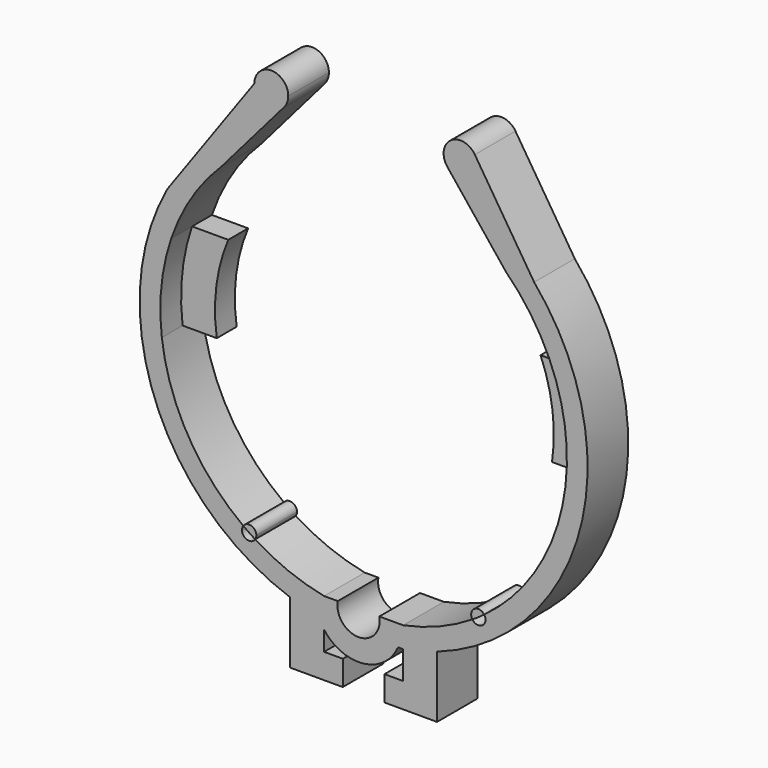
from build123d import *

# Parameters (mm, degrees)
F1_DEPTH = 4.5
F2_DEPTH = 2.2


with BuildPart() as f1:
    # F0 (on Front) → F1 (new body)
    with BuildSketch(Plane.XZ):
        with BuildLine():
            Line((-12.5982642878, 12.8562722799), (-17.3673227921, 9.5716989334))
            ThreePointArc((-17.3673227921, 9.5716989334), (-18.5128661298, -7.1073981948), (-6.5, -18.7347623801))
            ThreePointArc((-6.5, -18.7347623801), (-5.0153521077, -19.1856082696), (-3.5, -19.5189989866))
            Line((-3.5, -19.5189989866), (-3.5, -17.656443583))
            ThreePointArc((-3.5, -17.656443583), (-6.6633813431, -16.7212245089), (-9.6029714558, -15.2244191751))
            ThreePointArc((-9.6029714558, -15.2244191751), (-10.4915008811, -15.4010270522), (-10.6524086102, -14.5095206951))
            ThreePointArc((-10.6524086102, -14.5095206951), (-15.5351423919, -9.0917188069), (-17.8673478305, -2.1812568633))
            ThreePointArc((-17.8673478305, -2.1812568633), (-17.9030269403, 1.8659116739), (-17.033561821, 5.8187431367))
            ThreePointArc((-17.033561821, 5.8187431367), (-15.2280328258, 9.5972400332), (-12.5982642878, 12.8562722799))
        make_face()
        with BuildLine():
            Line((-9.6738959998, 20.2858578414), (-17.3673227921, 9.5716989334))
            Line((-17.3673227921, 9.5716989334), (-12.5982642878, 12.8562722799))
            Line((-12.5982642878, 12.8562722799), (-7.0377798874, 19.3064497655))
            ThreePointArc((-7.0377798874, 19.3064497655), (-8.696306677, 18.8797685539), (-9.6738959998, 20.2858578414))
        make_face()
        with BuildLine():
            ThreePointArc((-3.5, -19.5189989866), (-5.0153521077, -19.1856082696), (-6.5, -18.7347623801))
            Line((-6.5, -18.7347623801), (-6.5, -24.2152123027))
            Line((-6.5, -24.2152123027), (-1.8481902329, -24.2152123027))
            Line((-1.8481902329, -24.2152123027), (-1.8312213279, -22.0041828084))
            Line((-1.8312213279, -22.0041828084), (-3.5, -22.0041828084))
            Line((-3.5, -22.0041828084), (-3.5, -20.2840574679))
            ThreePointArc((-3.5, -20.2840574679), (-3.7451179805, -19.9145035902), (-3.945689667, -19.5189989866))
            Line((-3.945689667, -19.5189989866), (-3.5, -19.5189989866))
        make_face()
        with BuildLine():
            ThreePointArc((-6.6738959998, 20.2858578414), (-8.1738959998, 21.7858578414), (-9.6738959998, 20.2858578414))
            ThreePointArc((-9.6738959998, 20.2858578414), (-8.696306677, 18.8797685539), (-7.0377798874, 19.3064497655))
            ThreePointArc((-7.0377798874, 19.3064497655), (-6.7678067123, 19.7634471641), (-6.6738959998, 20.2858578414))
        make_face()
        with BuildLine():
            Line((-3.5, -17.656443583), (-3.5, -19.5189989866))
            Line((-3.5, -19.5189989866), (-3.5, -20.2840574679))
            ThreePointArc((-3.5, -20.2840574679), (-0.0064092924, -21.7831240851), (3.0474594497, -19.5189989866))
            Line((3.0474594497, -19.5189989866), (3.5, -19.5189989866))
            Line((3.5, -19.5189989866), (3.5, -17.656443583))
            Line((3.5, -17.656443583), (3.3503894936, -17.656443583))
            Line((3.3503894936, -17.656443583), (2.321347558, -17.656443583))
            Line((2.321347558, -17.656443583), (1.3912129293, -17.656443583))
            ThreePointArc((1.3912129293, -17.656443583), (-0.4491151087, -19.8654973153), (-2.2894431467, -17.656443583))
            Line((-2.2894431467, -17.656443583), (-2.854652442, -17.656443583))
            Line((-2.854652442, -17.656443583), (-3.5, -17.656443583))
        make_face()
        with BuildLine():
            Line((-3.5, -20.2840574679), (-3.5, -19.5189989866))
            Line((-3.5, -19.5189989866), (-3.945689667, -19.5189989866))
            ThreePointArc((-3.945689667, -19.5189989866), (-3.7451179805, -19.9145035902), (-3.5, -20.2840574679))
        make_face()
        with BuildLine():
            ThreePointArc((6.5, -18.7347623801), (5.0153521077, -19.1856082696), (3.5, -19.5189989866))
            Line((3.5, -19.5189989866), (3.5, -22.0041828084))
            Line((3.5, -22.0041828084), (1.8481902329, -22.0041828084))
            Line((1.8481902329, -22.0041828084), (1.8312213279, -24.2152123027))
            Line((1.8312213279, -24.2152123027), (6.5, -24.2152123027))
            Line((6.5, -24.2152123027), (6.5, -18.7347623801))
        make_face()
        with BuildLine():
            Line((3.5, -17.656443583), (3.5, -19.5189989866))
            ThreePointArc((3.5, -19.5189989866), (5.0153521077, -19.1856082696), (6.5, -18.7347623801))
            ThreePointArc((6.5, -18.7347623801), (19.1342526058, -5.2078497151), (15.0982642878, 12.8562722799))
            Line((15.0982642878, 12.8562722799), (12.5982642878, 12.8562722799))
            ThreePointArc((12.5982642878, 12.8562722799), (15.2280328258, 9.5972400332), (17.033561821, 5.8187431367))
            ThreePointArc((17.033561821, 5.8187431367), (17.9030269403, 1.8659116739), (17.8673478305, -2.1812568633))
            ThreePointArc((17.8673478305, -2.1812568633), (15.5430874553, -9.0781293423), (10.6777704031, -14.4908667518))
            ThreePointArc((10.6777704031, -14.4908667518), (10.7649831427, -14.665553176), (10.795, -14.8584790608))
            ThreePointArc((10.795, -14.8584790608), (10.3422246395, -15.4667710801), (9.6295852574, -15.2075996715))
            ThreePointArc((9.6295852574, -15.2075996715), (6.6780020503, -16.7153907707), (3.5, -17.656443583))
        make_face()
        with BuildLine():
            Line((12.5982642878, 12.8562722799), (15.0982642878, 12.8562722799))
            Line((15.0982642878, 12.8562722799), (9.8459355165, 21.0923907272))
            ThreePointArc((9.8459355165, 21.0923907272), (10.0211981842, 20.7059334899), (10.0812202505, 20.2858578414))
            ThreePointArc((10.0812202505, 20.2858578414), (9.0773524967, 18.8702827659), (7.4094165247, 19.3494412523))
            Line((7.4094165247, 19.3494412523), (12.5982642878, 12.8562722799))
        make_face()
        with BuildLine():
            ThreePointArc((10.0812202505, 20.2858578414), (10.0211981842, 20.7059334899), (9.8459355165, 21.0923907272))
            ThreePointArc((9.8459355165, 21.0923907272), (7.7085081809, 21.5058470395), (7.4094165247, 19.3494412523))
            ThreePointArc((7.4094165247, 19.3494412523), (9.0773524967, 18.8702827659), (10.0812202505, 20.2858578414))
        make_face()
    extrude(amount=F1_DEPTH)


with BuildPart() as f1b:
    # F0 (on Front) → F1, piece 2 (new body)
    with BuildSketch(Plane.XZ):
        with BuildLine():
            ThreePointArc((-10.6524086102, -14.5095206951), (-10.1339960215, -14.8762268279), (-9.6029714558, -15.2244191751))
            ThreePointArc((-9.6029714558, -15.2244191751), (-9.5255448734, -15.0579194266), (-9.4989960215, -14.8762268279))
            ThreePointArc((-9.4989960215, -14.8762268279), (-9.9415992879, -14.2710751966), (-10.6524086102, -14.5095206951))
        make_face()
    extrude(amount=F1_DEPTH)


with BuildPart() as f1c:
    # F0 (on Front) → F1, piece 3 (new body)
    with BuildSketch(Plane.XZ):
        with BuildLine():
            ThreePointArc((10.6777704031, -14.4908667518), (9.8015777778, -14.3343049384), (9.6295852574, -15.2075996715))
            ThreePointArc((9.6295852574, -15.2075996715), (10.16, -14.8584790608), (10.6777704031, -14.4908667518))
        make_face()
    extrude(amount=F1_DEPTH)


with BuildPart() as f2:
    # F0 (on Front) → F2 (new body)
    with BuildSketch(Plane.XZ):
        with BuildLine():
            Line((-13.8254196431, 5.8187431367), (-17.033561821, 5.8187431367))
            ThreePointArc((-17.033561821, 5.8187431367), (-17.9030269403, 1.8659116739), (-17.8673478305, -2.1812568633))
            Line((-17.8673478305, -2.1812568633), (-14.8405565427, -2.1812568633))
            ThreePointArc((-14.8405565427, -2.1812568633), (-14.8806769897, 1.8882405378), (-13.8254196431, 5.8187431367))
        make_face()
    extrude(amount=F2_DEPTH)


with BuildPart() as f2b:
    # F0 (on Front) → F2, piece 2 (new body)
    with BuildSketch(Plane.XZ):
        with BuildLine():
            Line((14.8405565427, -2.1812568633), (17.8673478305, -2.1812568633))
            ThreePointArc((17.8673478305, -2.1812568633), (17.9030269403, 1.8659116739), (17.033561821, 5.8187431367))
            Line((17.033561821, 5.8187431367), (13.8254196431, 5.8187431367))
            ThreePointArc((13.8254196431, 5.8187431367), (14.8806769897, 1.8882405378), (14.8405565427, -2.1812568633))
        make_face()
    extrude(amount=F2_DEPTH)


solid = Compound([f1.part, f1b.part, f1c.part, f2.part, f2b.part])
